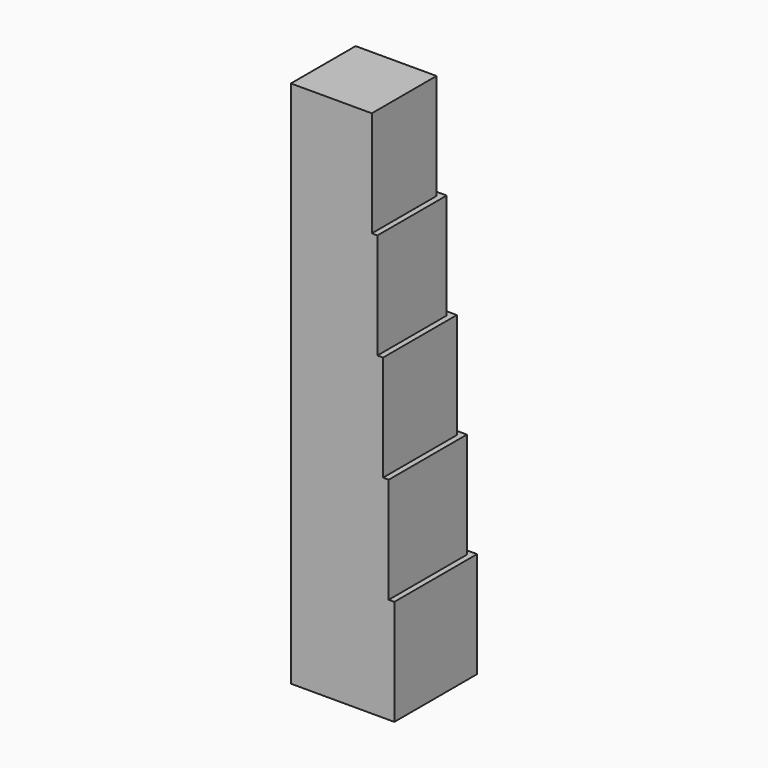
from build123d import *

# Parameters (mm, degrees)
F1_W      = 4.6609
F1_H      = 4.6609
F2_DEPTH  = 4.7625
F3_W      = 4.4069
F3_H      = 4.4069
F4_DEPTH  = 4.7625
F5_W      = 4.1529
F5_H      = 4.1529
F6_DEPTH  = 4.7625
F7_W      = 3.8989
F7_H      = 3.8989
F8_DEPTH  = 4.7625
F9_W      = 3.6449
F9_H      = 3.6449
F10_DEPTH = 4.7625


# Not quite as in the source:
# - a variable given as a bare number and used for a length is read in inches; the dataset says mm whatever the document's units were


with BuildPart() as f2:
    # F1 (on Top) → F2 (new body)
    with BuildSketch(Plane.XY):
        with Locations((2.33045, 2.33045)):
            Rectangle(F1_W, F1_H)
    extrude(amount=F2_DEPTH)

    # F3 (on face) → F4 (join)
    with BuildSketch(Plane.XY.offset(4.7625)):
        with Locations((2.20345, 2.20345)):
            Rectangle(F3_W, F3_H)
    extrude(amount=F4_DEPTH)

    # F5 (on face) → F6 (join)
    with BuildSketch(Plane.XY.offset(9.525)):
        with Locations((2.07645, 2.07645)):
            Rectangle(F5_W, F5_H)
    extrude(amount=F6_DEPTH)

    # F7 (on face) → F8 (join)
    with BuildSketch(Plane.XY.offset(14.2875)):
        with Locations((1.94945, 1.94945)):
            Rectangle(F7_W, F7_H)
    extrude(amount=F8_DEPTH)

    # F9 (on face) → F10 (join)
    with BuildSketch(Plane.XY.offset(19.05)):
        with Locations((1.82245, 1.82245)):
            Rectangle(F9_W, F9_H)
    extrude(amount=F10_DEPTH)


solid = f2.part
